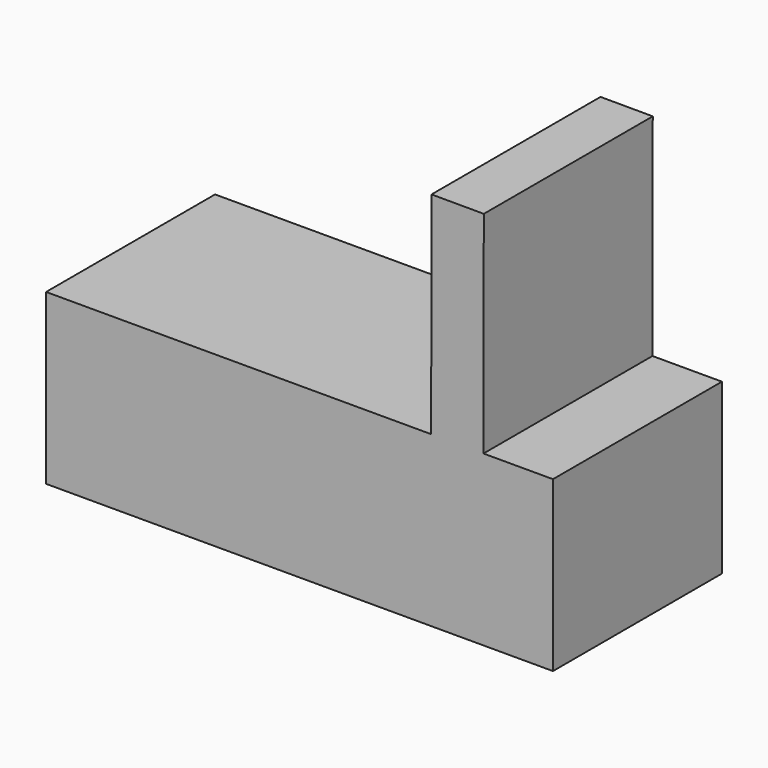
from build123d import *

# Parameters (mm, degrees)
F1_DEPTH = 25
F2_DEPTH = 25


# Not quite as in the source:
# - ends of sketch curves that miss each other by under 0.0002 mm in the source are joined
# - the dataset's text gives a spline's control points without its knots; the knots are read off the source's solid


with BuildPart() as f1:
    # F0 (on Front) → F1 (new body)
    with BuildSketch(Plane.XZ):
        with BuildLine():
            Line((-22.0594022245, 9.6566297112), (-67.6395371556, 9.6566297112))
            Line((-67.6395371556, 9.6566297112), (-67.6395371556, -10.3433702888))
            Line((-67.6395371556, -10.3433702888), (-7.6395371556, -10.3433702888))
            Line((-7.6395371556, -10.3433702888), (-7.6395371556, 9.6566297112))
            Line((-7.6395371556, 9.6566297112), (-15.8638085328, 9.6566297112))
            add(Edge.make_bspline(
                [(-15.872090736, 9.6453477446), (-15.8693299564, 9.6491085329), (-15.866569222, 9.6528691885), (-15.8638085328, 9.6566297112)],
                knots=[0.0211094133, 0.0211094133, 0.0211094133, 0.0211094133, 0.0211910509, 0.0211910509, 0.0211910509, 0.0211910509], degree=3))
            Line((-15.872090736, 9.6453477446), (-22.0594022245, 9.6566297112))
        make_face()
    extrude(amount=F1_DEPTH)

    # F2 (add): a face of the model
    f2_faces = [f1.faces().sort_by_distance(p)[0] for p in [
        (-18.9657464803, -12.5, 9.6509887279),
    ]]
    extrude(f2_faces, amount=F2_DEPTH)


solid = f1.part
